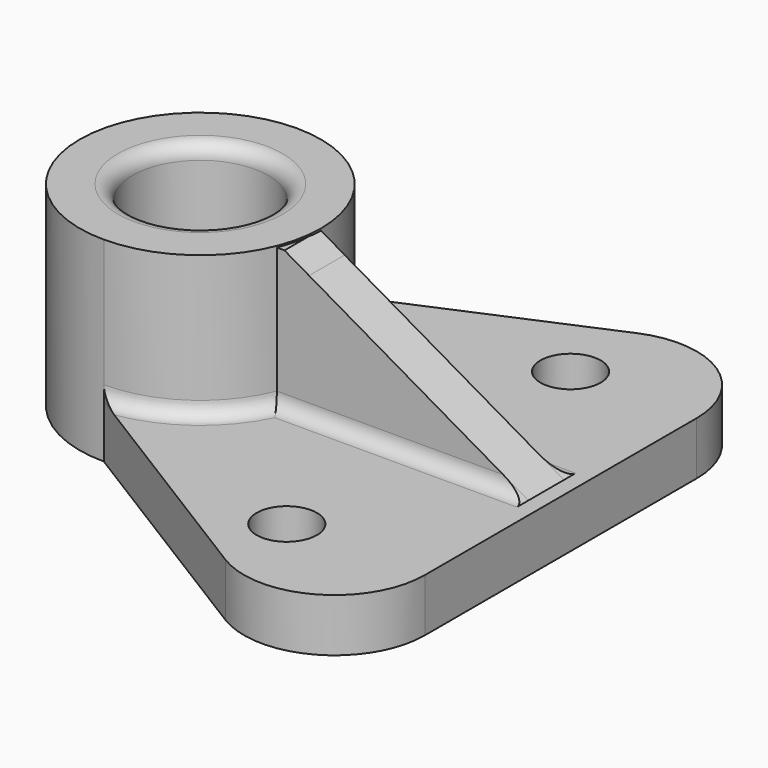
from build123d import *

# Parameters (mm, degrees)
F0_R         = 14.2875
F1_DEPTH     = 41.148
F0_R_2       = 6.35
F2_DEPTH     = 11.176
F4_DEPTH     = 26.67
F6_DEPTH     = 25.4
F7_DEPTH     = 9.398
F8_T4_DEPTH  = 66.4333664876
F8_T9_ANGLE  = 124.391277417
F8_T14_DEPTH = 68.2254329645
F8_T19_ANGLE = 102.7340831682


# Not quite as in the source:
# - a fillet or chamfer that OpenCascade refuses, or shapes differently, is made with other operations: its cross-section is extruded or revolved along the edge and cut away or added


with BuildPart() as f1:
    # F0 (on Top) → F1 (new body)
    with BuildSketch(Plane.XY):
        with BuildLine():
            ThreePointArc((0, -25.4), (17.9605122421, -17.9605122421), (25.4, 0))
            ThreePointArc((25.4, 0), (17.9605122421, 17.9605122421), (0, 25.4))
            ThreePointArc((0, 25.4), (-25.4, 0), (0, -25.4))
        make_face()
        Circle(F0_R, mode=Mode.SUBTRACT)
    extrude(amount=F1_DEPTH)

    # F0 (on Top) → F2 (join)
    with BuildSketch(Plane.XY):
        with BuildLine():
            ThreePointArc((0, 25.4), (17.9605122421, 17.9605122421), (25.4, 0))
            ThreePointArc((25.4, 0), (17.9605122421, -17.9605122421), (0, -25.4))
            Line((0, -25.4), (50.8, -56.9271389808))
            ThreePointArc((50.8, -56.9271389808), (70.1065291687, -57.388260775), (79.8953664876, -40.740937693))
            Line((79.8953664876, -40.740937693), (79.8953664876, 30.8181623129))
            ThreePointArc((79.8953664876, 30.8181623129), (71.3237376894, 46.7274752131), (53.3225332112, 48.3198616445))
            Line((53.3225332112, 48.3198616445), (0, 25.4))
        make_face()
        with Locations((50.8, -40.740937693)):
            Circle(F0_R_2, mode=Mode.SUBTRACT)
        with Locations((53.3225332112, 30.8181623129)):
            Circle(F0_R_2, mode=Mode.SUBTRACT)
    extrude(amount=F2_DEPTH)

    # F3 (on face) → F4 (join)
    with BuildSketch(Plane.XY.offset(11.176)):
        with BuildLine():
            Line((76.5933664876, -9.3715246767), (76.5933664876, 0))
            Line((76.5933664876, 0), (25.4, 0))
            ThreePointArc((25.4, 0), (24.9479609536, -4.77066497), (23.6079335232, -9.3715246767))
            Line((23.6079335232, -9.3715246767), (76.5933664876, -9.3715246767))
        make_face()
    extrude(amount=F4_DEPTH)

    # F5 (on face) → F6 (cut)
    with BuildSketch(Plane.XZ.offset(9.3715246767)):
        Polygon((76.5933664876, 37.846), (30.3995714498, 37.846), (76.5933664876, 11.176), align=None)
    extrude(amount=-F6_DEPTH, mode=Mode.SUBTRACT)

    # F5 (on face) → F7 (join)
    with BuildSketch(Plane.XZ.offset(9.3715246767)):
        Polygon((30.3995714498, 37.846), (25.2215964692, 40.8355052489), (23.6079335232, 40.8355052489), (23.6079335232, 37.846), align=None)
    extrude(amount=-F7_DEPTH)

    # F8: fillet of radius 3.048 on 5 edges, made by hand


with BuildPart() as f8_tool2:
    # F8_s3 → F8_t4 (new body)
    with BuildSketch(Plane.YZ.offset(84.2133664876)):
        with BuildLine():
            ThreePointArc((0, 14.224), (0.8927385309, 12.0687385309), (3.048, 11.176))
            Line((3.048, 11.176), (0, 11.176))
            Line((0, 11.176), (0, 14.224))
        make_face()
    extrude(amount=-F8_T4_DEPTH)

    split(bisect_by=Plane(origin=(23.9876915783, 0, 41.5479005698), x_dir=(0, 1, 0), z_dir=(-0.5, 0, -0.8660254038)), keep=Keep.TOP)


with BuildPart() as f1_1:
    add(f1.part)

    # F8_t1: union F8_tool2
    add(f8_tool2.part)


with BuildPart() as f8_tool7:
    # F8_s8 → F8_t9 (revolve)
    with BuildSketch(Plane(origin=(0, 0, 0), x_dir=(0, 0, 1), z_dir=(-0.2956353345, -0.9553008683, 0))):
        with BuildLine():
            ThreePointArc((14.224, -25.4), (12.0687385309, -26.2927385309), (11.176, -28.448))
            Line((11.176, -28.448), (11.176, -25.4))
            Line((11.176, -25.4), (14.224, -25.4))
        make_face()
    revolve(axis=Axis((0, 0, 11.176), (0, 0, 1)), revolution_arc=F8_T9_ANGLE)

    split(bisect_by=Plane(origin=(-9.2152137271, 21.4389836917, 0), x_dir=(0, 0, 1), z_dir=(0.3948993846, -0.9187243744, 0)), keep=Keep.TOP)


with BuildPart() as f1_2:
    add(f1_1.part)

    # F8_t6: union F8_tool7
    add(f8_tool7.part)


with BuildPart() as f8_tool12:
    # F8_s13 → F8_t14 (new body)
    with BuildSketch(Plane.YZ.offset(15.9879335232)):
        with BuildLine():
            ThreePointArc((-9.3715246767, 14.224), (-10.2642632076, 12.0687385309), (-12.4195246767, 11.176))
            Line((-12.4195246767, 11.176), (-9.3715246767, 11.176))
            Line((-9.3715246767, 11.176), (-9.3715246767, 14.224))
        make_face()
    extrude(amount=F8_T14_DEPTH)

    split(bisect_by=Plane(origin=(23.9876915783, 0, 41.5479005698), x_dir=(0, 1, 0), z_dir=(-0.5, 0, -0.8660254038)), keep=Keep.TOP)


with BuildPart() as f1_3:
    add(f1_2.part)

    # F8_t11: union F8_tool12
    add(f8_tool12.part)


with BuildPart() as f8_tool17:
    # F8_s18 → F8_t19 (revolve)
    with BuildSketch(Plane(origin=(0, 0, 0), x_dir=(0, 0, 1), z_dir=(-0.9553159496, 0.2955865973, 0))):
        with BuildLine():
            ThreePointArc((14.224, -25.4), (12.0687385309, -26.2927385309), (11.176, -28.448))
            Line((11.176, -28.448), (11.176, -25.4))
            Line((11.176, -25.4), (14.224, -25.4))
        make_face()
    revolve(axis=Axis((0, 0, 11.176), (0, 0, 1)), revolution_arc=F8_T19_ANGLE)

    split(bisect_by=Plane(origin=(-11.3803201385, -18.3372256958, 0), x_dir=(0, 0, 1), z_dir=(0.5273158261, 0.8496693589, 0)), keep=Keep.TOP)


with BuildPart() as f1_4:
    add(f1_3.part)

    # F8_t16: union F8_tool17
    add(f8_tool17.part)

    # F8_s21 → F8_t22 (revolve, cut)
    with BuildSketch(Plane.XZ):
        with BuildLine():
            ThreePointArc((17.3355, 41.148), (15.1802385309, 40.2552614691), (14.2875, 38.1))
            Line((14.2875, 38.1), (14.2875, 41.148))
            Line((14.2875, 41.148), (17.3355, 41.148))
        make_face()
    revolve(axis=Axis((0, 0, 41.148), (0, 0, 1)), mode=Mode.SUBTRACT)


solid = f1_4.part
